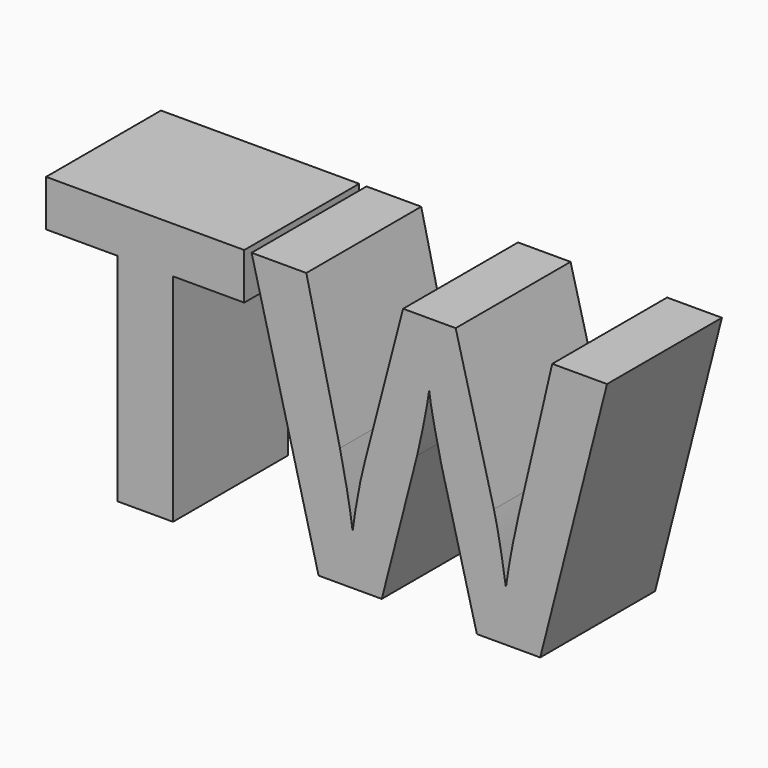
from build123d import *

# Parameters (mm, degrees)
F0_TEXT_SIZE = 65.0119107579
F1_DEPTH     = 25.4


# Not quite as in the source:
# - a feature names something its author has since deleted; it is built from what else it names
# - Text() gives the source's letters only with a copy of the font that has no kerning and outlines rounded to 1/6400 em; it was checked with that copy


with BuildPart() as f1:
    # F0 (on Front) → F1 (new body)
    with BuildSketch(Plane.XZ):
        with Locations((-75.3835737705, 4.445000086)):
            Text('TW', F0_TEXT_SIZE, font='Open Sans', font_style=FontStyle.BOLD, text_align=(TextAlign.LEFT, TextAlign.BOTTOM))
    extrude(amount=F1_DEPTH)


solid = f1.part
